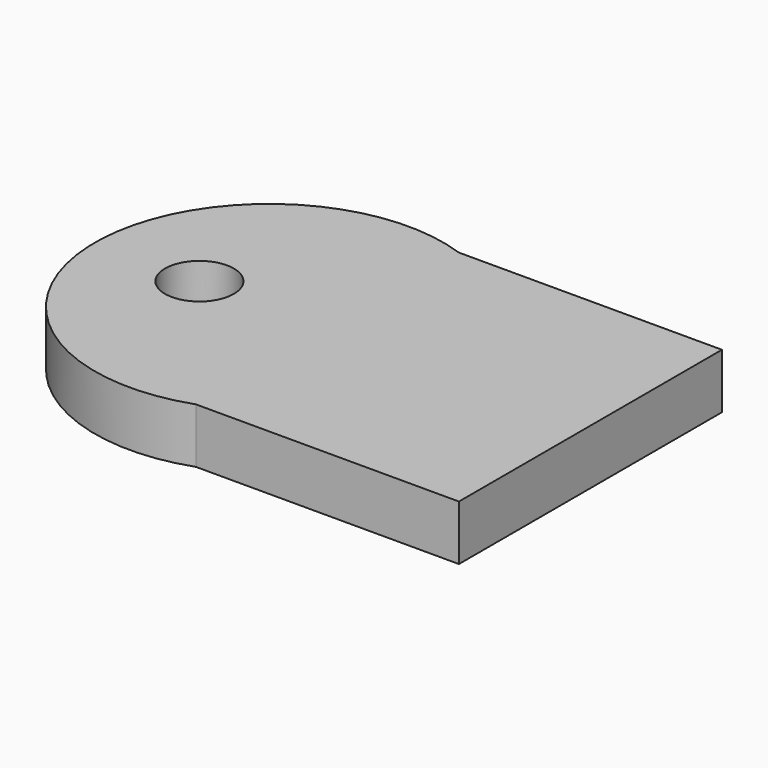
from build123d import *

# Parameters (mm, degrees)
F0_R     = 12.5
F1_DEPTH = 20


# Not quite as in the source:
# - a feature names something its author has since deleted; it is built from what else it names


with BuildPart() as f1:
    # F0 (on Top) → F1 (new body)
    with BuildSketch(Plane.XY):
        with BuildLine():
            Line((21.7014607042, 59.7112393002), (-73.8888888889, 59.7112393002))
            ThreePointArc((-73.8888888889, 59.7112393002), (-158.3333333333, 0), (-73.8888888889, -59.7112393002))
            Line((-73.8888888889, -59.7112393002), (21.7014607042, -59.7112393002))
            Line((21.7014607042, -59.7112393002), (21.7014607042, 59.7112393002))
        make_face()
        with Locations((-120.3333333333, 0)):
            Circle(F0_R, mode=Mode.SUBTRACT)
    extrude(amount=F1_DEPTH)


solid = f1.part
